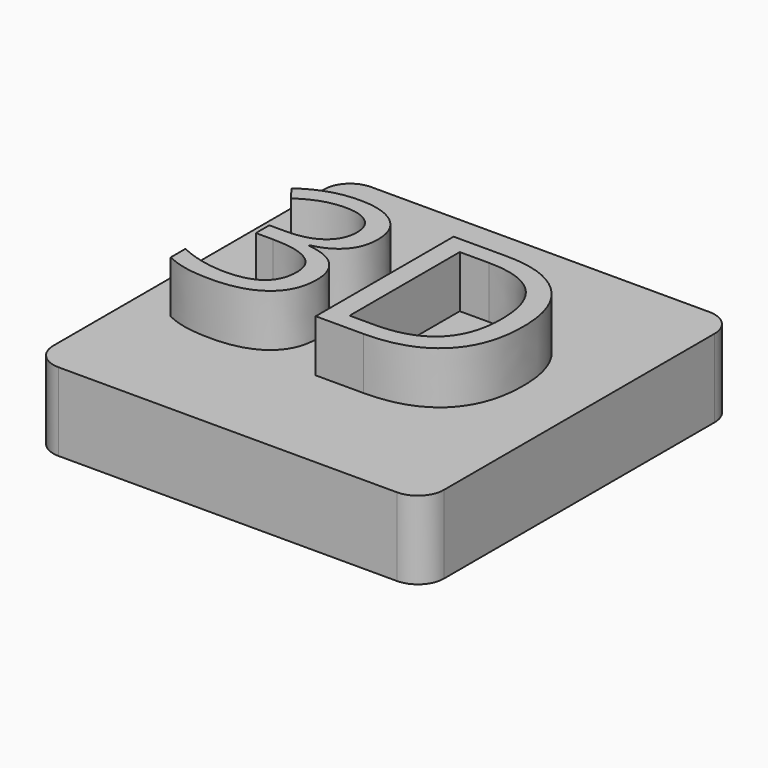
from build123d import *

# Parameters (mm, degrees)
F1_DEPTH     = 3
F2_TEXT_SIZE = 9.2738104286
F3_DEPTH     = 2


# Not quite as in the source:
# - Text() gives the source's letters only with a copy of the font that has no kerning and outlines rounded to 1/6400 em; it was checked with that copy


with BuildPart() as f1:
    # F0 (on Top) → F1 (new body)
    with BuildSketch(Plane.XY):
        with BuildLine():
            Line((-6.5, -7.5), (6.5, -7.5))
            ThreePointArc((6.5, -7.5), (7.2071067812, -7.2071067812), (7.5, -6.5))
            Line((7.5, -6.5), (7.5, 6.5))
            ThreePointArc((7.5, 6.5), (7.2071067812, 7.2071067812), (6.5, 7.5))
            Line((6.5, 7.5), (-6.5, 7.5))
            ThreePointArc((-6.5, 7.5), (-7.2071067812, 7.2071067812), (-7.5, 6.5))
            Line((-7.5, 6.5), (-7.5, -6.5))
            ThreePointArc((-7.5, -6.5), (-7.2071067812, -7.2071067812), (-6.5, -7.5))
        make_face()
    extrude(amount=F1_DEPTH)

    # F2 (on face) → F3 (join)
    with BuildSketch(Plane.XY.offset(3)):
        with Locations((-6.3612041995, -3.0922885053)):
            Text('3D', F2_TEXT_SIZE, font='Open Sans', text_align=(TextAlign.LEFT, TextAlign.BOTTOM))
    extrude(amount=F3_DEPTH)


solid = f1.part
